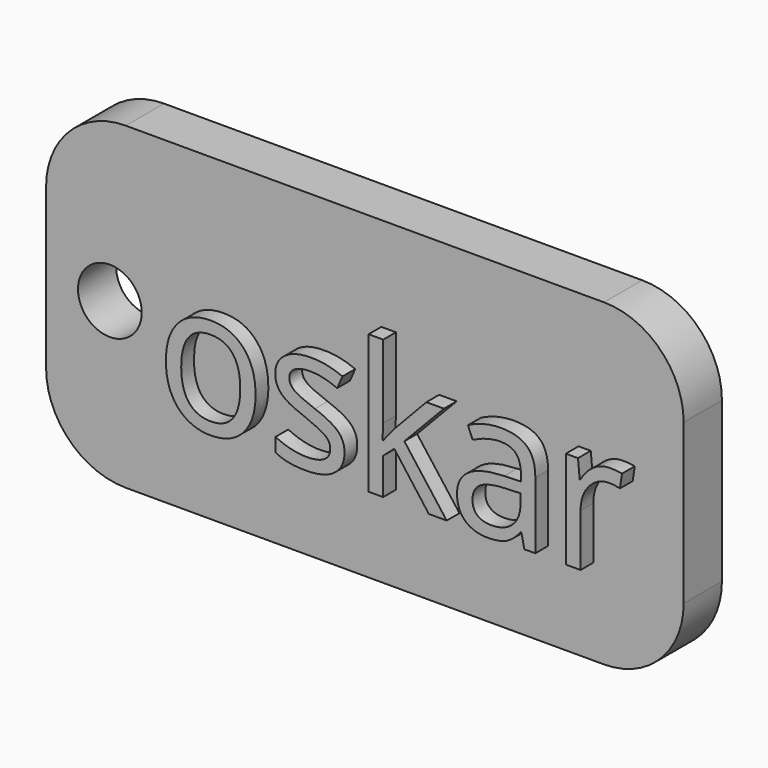
from build123d import *

# Parameters (mm, degrees)
F1_DEPTH     = 3
F2_R         = 2
F3_DEPTH     = 5
F4_TEXT_SIZE = 11.4462859187
F5_DEPTH     = 1


# Not quite as in the source:
# - Text() gives the source's letters only with a copy of the font that has no kerning and outlines rounded to 1/6400 em; it was checked with that copy


with BuildPart() as f1:
    # F0 (on Front) → F1 (new body)
    with BuildSketch(Plane.XZ):
        with BuildLine():
            Line((35, 20), (5, 20))
            ThreePointArc((5, 20), (1.4644660941, 18.5355339059), (0, 15))
            Line((0, 15), (0, 5))
            ThreePointArc((0, 5), (1.4644660941, 1.4644660941), (5, 0))
            Line((5, 0), (35, 0))
            ThreePointArc((35, 0), (38.5355339059, 1.4644660941), (40, 5))
            Line((40, 5), (40, 15))
            ThreePointArc((40, 15), (38.5355339059, 18.5355339059), (35, 20))
        make_face()
    extrude(amount=F1_DEPTH)

    # F2 (on Front) → F3 (cut)
    with BuildSketch(Plane.XZ):
        with Locations((4, 10)):
            Circle(F2_R)
    extrude(amount=F3_DEPTH, mode=Mode.SUBTRACT)

    # F4 (on face) → F5 (join)
    with BuildSketch(Plane.XZ.offset(3)):
        with Locations((7.6732230064, 5.4034209818)):
            Text('oskar', F4_TEXT_SIZE, font='Open Sans', text_align=(TextAlign.LEFT, TextAlign.BOTTOM))
    extrude(amount=F5_DEPTH)


solid = f1.part
